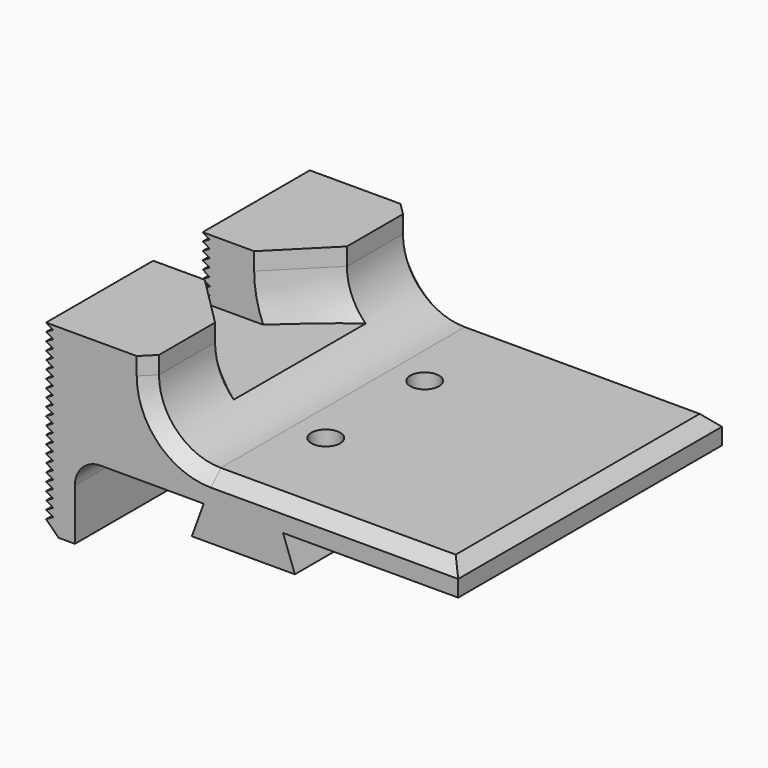
from build123d import *

# Parameters (mm, degrees)
F1_DEPTH     = 10.16
F2_W         = 3.81
F2_H         = 3.81
F3_DEPTH     = 25.4
F4_R         = 1.5875
F5_T4_DEPTH  = 20.32
F5_T10_DEPTH = 20.32
F5_T16_DEPTH = 20.32
F5_T23_DEPTH = 20.32
F5_T29_DEPTH = 20.32
F6_SIZE      = 3.175
F7_SIZE      = 0.762
F8_SIZE      = 0.762
F10_D        = 1.778
F12_DEPTH    = 25.4


# Not quite as in the source:
# - a fillet or chamfer that OpenCascade refuses, or shapes differently, is made with other operations: its cross-section is extruded or revolved along the edge and cut away or added


with BuildPart() as f1:
    # F0 (on Front) → F1 (new body, symmetric)
    with BuildSketch(Plane.XZ):
        Polygon((-8.382, 0), (-0.4445, 0), (-1.1748426721, -2.0066), (5.1751573279, -2.0066), (4.4448146558, 0), (15.24, 0), (15.24, 1.778), (-3.81, 1.778), (-3.81, 6.6675), (-10.16, 6.6675), (-10.16, -4.7625), (-8.382, -4.7625), align=None)
    extrude(amount=F1_DEPTH, both=True)

    # F2 (on face) → F3 (cut)
    with BuildSketch(Plane(origin=(-10.16, 0, 0), x_dir=(0, -1, 0), z_dir=(-1, 0, 0))):
        with Locations((0, 4.7625)):
            Rectangle(F2_W, F2_H)
    extrude(amount=-F3_DEPTH, mode=Mode.SUBTRACT)

    # F4
    f4_edges = [f1.edges().sort_by_distance(p)[0] for p in [
        (-8.382, 0, 0),
    ]]
    fillet(f4_edges, radius=F4_R)

    # F5: fillet of radius 3.81 on 1 edges, made by hand


with BuildPart() as f5_tool2:
    # F5_s3 → F5_t4 (new body)
    with BuildSketch(Plane.XZ.offset(10.16)):
        with BuildLine():
            ThreePointArc((-3.81, 5.588), (-2.6940768363, 2.8939231637), (0, 1.778))
            Line((0, 1.778), (-3.81, 1.778))
            Line((-3.81, 1.778), (-3.81, 5.588))
        make_face()
    extrude(amount=-F5_T4_DEPTH)

    split(bisect_by=Plane.XZ.offset(1.905), keep=Keep.TOP)

    split(bisect_by=Plane.XY.offset(2.8575), keep=Keep.TOP)


with BuildPart() as f1_1:
    add(f1.part)

    # F5_t1: union F5_tool2
    add(f5_tool2.part)


with BuildPart() as f5_tool8:
    # F5_s9 → F5_t10 (new body)
    with BuildSketch(Plane.XZ.offset(10.16)):
        with BuildLine():
            ThreePointArc((-3.81, 5.588), (-2.6940768363, 2.8939231637), (0, 1.778))
            Line((0, 1.778), (-3.81, 1.778))
            Line((-3.81, 1.778), (-3.81, 5.588))
        make_face()
    extrude(amount=-F5_T10_DEPTH)

    split(bisect_by=Plane.XZ.offset(1.905), keep=Keep.TOP)

    split(bisect_by=Plane.XY.offset(2.8575), keep=Keep.BOTTOM)


with BuildPart() as f1_2:
    add(f1_1.part)

    # F5_t7: union F5_tool8
    add(f5_tool8.part)


with BuildPart() as f5_tool14:
    # F5_s15 → F5_t16 (new body)
    with BuildSketch(Plane.XZ.offset(10.16)):
        with BuildLine():
            ThreePointArc((-3.81, 5.588), (-2.6940768363, 2.8939231637), (0, 1.778))
            Line((0, 1.778), (-3.81, 1.778))
            Line((-3.81, 1.778), (-3.81, 5.588))
        make_face()
    extrude(amount=-F5_T16_DEPTH)

    split(bisect_by=Plane.XZ.offset(1.905), keep=Keep.BOTTOM)

    split(bisect_by=Plane.XY.offset(2.8575), keep=Keep.BOTTOM)

    split(bisect_by=Plane.XZ.offset(-1.905), keep=Keep.TOP)


with BuildPart() as f1_3:
    add(f1_2.part)

    # F5_t13: union F5_tool14
    add(f5_tool14.part)


with BuildPart() as f5_tool21:
    # F5_s22 → F5_t23 (new body)
    with BuildSketch(Plane.XZ.offset(10.16)):
        with BuildLine():
            ThreePointArc((-3.81, 5.588), (-2.6940768363, 2.8939231637), (0, 1.778))
            Line((0, 1.778), (-3.81, 1.778))
            Line((-3.81, 1.778), (-3.81, 5.588))
        make_face()
    extrude(amount=-F5_T23_DEPTH)

    split(bisect_by=Plane.XY.offset(2.8575), keep=Keep.TOP)

    split(bisect_by=Plane.XZ.offset(-1.905), keep=Keep.BOTTOM)


with BuildPart() as f1_4:
    add(f1_3.part)

    # F5_t20: union F5_tool21
    add(f5_tool21.part)


with BuildPart() as f5_tool27:
    # F5_s28 → F5_t29 (new body)
    with BuildSketch(Plane.XZ.offset(10.16)):
        with BuildLine():
            ThreePointArc((-3.81, 5.588), (-2.6940768363, 2.8939231637), (0, 1.778))
            Line((0, 1.778), (-3.81, 1.778))
            Line((-3.81, 1.778), (-3.81, 5.588))
        make_face()
    extrude(amount=-F5_T29_DEPTH)

    split(bisect_by=Plane.XY.offset(2.8575), keep=Keep.BOTTOM)

    split(bisect_by=Plane.XZ.offset(-1.905), keep=Keep.BOTTOM)


with BuildPart() as f1_5:
    add(f1_4.part)

    # F5_t26: union F5_tool27
    add(f5_tool27.part)

    # F6
    f6_edges = [f1_5.edges().sort_by_distance(p)[0] for p in [
        (-3.509976, -1.905, 4.106052),
        (-3.509976, 1.905, 4.106052),
    ]]
    chamfer(f6_edges, length=F6_SIZE)

    # F7
    f7_edges = [f1_5.edges().sort_by_distance(p)[0] for p in [
        (-10.16, 0, -4.7625),
    ]]
    chamfer(f7_edges, length=F7_SIZE)

    # F8
    f8_edges = [f1_5.edges().sort_by_distance(p)[0] for p in [
        (-2.694077, -10.16, 2.893923),
        (7.62, -10.16, 1.778),
        (7.62, 10.16, 1.778),
        (15.24, 0, 1.778),
    ]]
    chamfer(f8_edges, length=F8_SIZE)

    # F10 (through all)
    with Locations(Plane(origin=(0, 0, -2.0066), x_dir=(1, 0, 0), z_dir=(0, 0, -1))):
        with Locations((2.0001573279, 3.81), (2.0001573279, -3.81)):
            Hole(F10_D / 2)

    # F11 (on face) → F12 (cut)
    with BuildSketch(Plane.XZ.offset(10.16)):
        Polygon((-10.16, -3.4925), (-10.16, -4.0005), (-9.7200590949, -3.7465), align=None)
        Polygon((-10.16, -2.9845), (-10.16, -3.4925), (-9.7200590949, -3.2385), align=None)
        Polygon((-10.16, -2.4765), (-10.16, -2.9845), (-9.7200590949, -2.7305), align=None)
        Polygon((-9.7200590949, -2.2225), (-10.16, -1.9685), (-10.16, -2.4765), align=None)
        Polygon((-9.7200590949, -1.7145), (-10.16, -1.4605), (-10.16, -1.9685), align=None)
        Polygon((-9.7200590949, -1.2065), (-10.16, -0.9525), (-10.16, -1.4605), align=None)
        Polygon((-9.7200590949, -0.6985), (-10.16, -0.4445), (-10.16, -0.9525), align=None)
        Polygon((-9.7200590949, -0.1905), (-10.16, 0.0635), (-10.16, -0.4445), align=None)
        Polygon((-9.7200590949, 0.3175), (-10.16, 0.5715), (-10.16, 0.0635), align=None)
        Polygon((-9.7200590949, 0.8255), (-10.16, 1.0795), (-10.16, 0.5715), align=None)
        Polygon((-9.7200590949, 1.3335), (-10.16, 1.5875), (-10.16, 1.0795), align=None)
        Polygon((-9.7200590949, 1.8415), (-10.16, 2.0955), (-10.16, 1.5875), align=None)
        Polygon((-9.7200590949, 2.3495), (-10.16, 2.6035), (-10.16, 2.0955), align=None)
        Polygon((-9.7200590949, 2.8575), (-10.16, 3.1115), (-10.16, 2.6035), align=None)
        Polygon((-9.7200590949, 3.3655), (-10.16, 3.6195), (-10.16, 3.1115), align=None)
        Polygon((-9.7200590949, 3.8735), (-10.16, 4.1275), (-10.16, 3.6195), align=None)
        Polygon((-9.7200590949, 4.3815), (-10.16, 4.6355), (-10.16, 4.1275), align=None)
        Polygon((-9.7200590949, 4.8895), (-10.16, 5.1435), (-10.16, 4.6355), align=None)
        Polygon((-9.7200590949, 5.3975), (-10.16, 5.6515), (-10.16, 5.1435), align=None)
        Polygon((-9.7200590949, 5.9055), (-10.16, 6.1595), (-10.16, 5.6515), align=None)
        Polygon((-10.16, 6.1595), (-9.7200590949, 6.4135), (-10.16, 6.6675), align=None)
    extrude(amount=-F12_DEPTH, mode=Mode.SUBTRACT)


solid = f1_5.part
